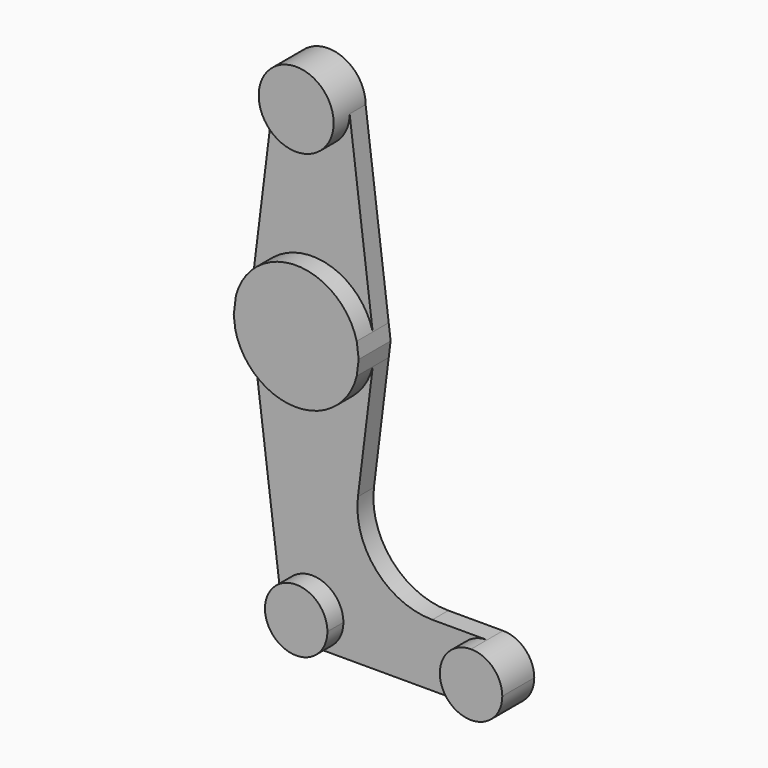
from build123d import *

# Parameters (mm, degrees)
F1_DEPTH = 2
F2_DEPTH = 4


with BuildPart() as f1:
    # F0 (on Front) → F1 (new body)
    with BuildSketch(Plane.XZ):
        with BuildLine():
            Line((6.0576923077, -18.4615384615), (3.75, 0))
            ThreePointArc((3.75, 0), (0, -3.75), (-3.75, 0))
            Line((-3.75, 0), (-6.0264121951, -18.3432392886))
            ThreePointArc((-6.0264121951, -18.3432392886), (0.0611823908, -13.75029947), (6.0576923077, -18.4615384615))
        make_face()
    extrude(amount=F1_DEPTH)


with BuildPart() as f1b:
    # F0 (on Front) → F1, piece 2 (new body)
    with BuildSketch(Plane.XZ):
        with BuildLine():
            Line((4.581416472, -33.451760418), (6.0605841498, -21.5270297191))
            ThreePointArc((6.0605841498, -21.5270297191), (-0.0567793323, -26.2497420833), (-6.0873278177, -21.416665112))
            Line((-6.0873278177, -21.416665112), (-3.1249885099, -44.9915257414))
            ThreePointArc((-3.1249885099, -44.9915257414), (0.0042371332, -41.8750028725), (3.125, -45))
            ThreePointArc((3.125, -45), (2.2097086912, -47.2097086912), (0, -48.125))
            Line((0, -48.125), (17.5, -48.125))
            ThreePointArc((17.5, -48.125), (14.375, -45), (17.5, -41.875))
            Line((17.5, -41.875), (12.0243748001, -41.875))
            ThreePointArc((12.0243748001, -41.875), (6.404130283, -39.3411707147), (4.581416472, -33.451760418))
        make_face()
    extrude(amount=F1_DEPTH)


with BuildPart() as f2:
    # F0 (on Front) → F2 (new body)
    with BuildSketch(Plane.XZ):
        with BuildLine():
            ThreePointArc((-3.75, 0), (0, -3.75), (3.75, 0))
            ThreePointArc((3.75, 0), (0, 3.75), (-3.75, 0))
        make_face()
    extrude(amount=F2_DEPTH)


with BuildPart() as f2b:
    # F0 (on Front) → F2, piece 2 (new body)
    with BuildSketch(Plane.XZ):
        with BuildLine():
            Line((6.25, -20), (6.0576923077, -18.4615384615))
            ThreePointArc((6.0576923077, -18.4615384615), (0.0611823908, -13.75029947), (-6.0264121951, -18.3432392886))
            Line((-6.0264121951, -18.3432392886), (-6.2485756833, -20.1334238753))
            Line((-6.2485756833, -20.1334238753), (-6.0873278177, -21.416665112))
            ThreePointArc((-6.0873278177, -21.416665112), (-0.0567793323, -26.2497420833), (6.0605841498, -21.5270297191))
            Line((6.0605841498, -21.5270297191), (6.25, -20))
        make_face()
    extrude(amount=F2_DEPTH)


with BuildPart() as f2c:
    # F0 (on Front) → F2, piece 3 (new body)
    with BuildSketch(Plane.XZ):
        with BuildLine():
            ThreePointArc((3.125, -45), (0.0042371332, -41.8750028725), (-3.1249885099, -44.9915257414))
            ThreePointArc((-3.1249885099, -44.9915257414), (-2.2127027657, -47.2067105544), (0, -48.125))
            ThreePointArc((0, -48.125), (2.2097086912, -47.2097086912), (3.125, -45))
        make_face()
    extrude(amount=F2_DEPTH)


with BuildPart() as f2d:
    # F0 (on Front) → F2, piece 4 (new body)
    with BuildSketch(Plane.XZ):
        with BuildLine():
            ThreePointArc((20.625, -45), (19.7097086912, -42.7902913088), (17.5, -41.875))
            ThreePointArc((17.5, -41.875), (14.375, -45), (17.5, -48.125))
            ThreePointArc((17.5, -48.125), (19.7097086912, -47.2097086912), (20.625, -45))
        make_face()
    extrude(amount=F2_DEPTH)


solid = Compound([f1.part, f1b.part, f2.part, f2b.part, f2c.part, f2d.part])
